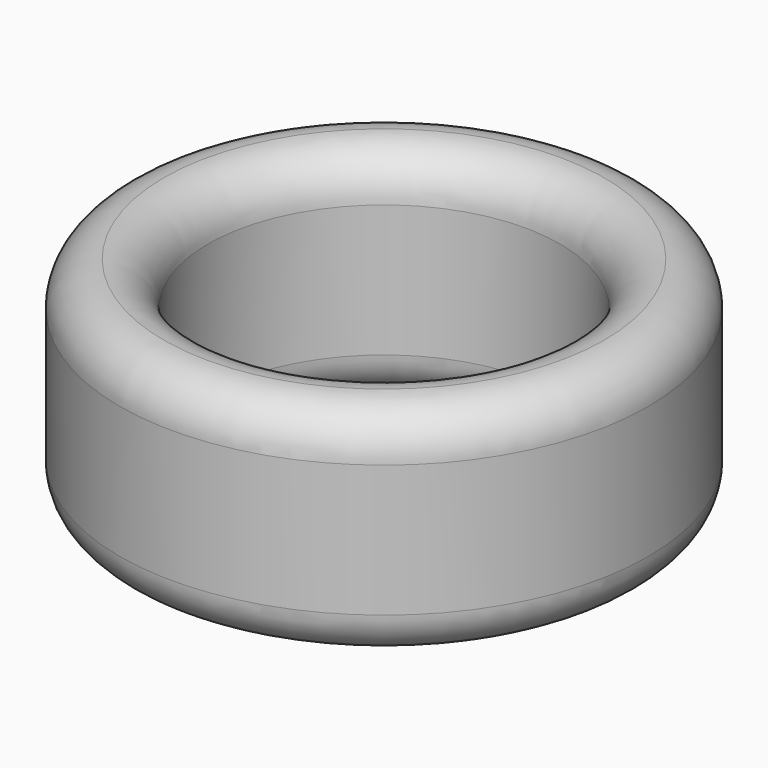
from build123d import *

# Parameters (mm, degrees)
F0_R     = 30
F0_R_2   = 20
F1_DEPTH = 25
F2_R     = 4.99999


# Not quite as in the source:
# - a fillet or chamfer is up to 0.001 mm smaller than in the source, because OpenCascade refuses the exact size


with BuildPart() as f1:
    # F0 (on Top) → F1 (new body)
    with BuildSketch(Plane.XY):
        Circle(F0_R)
        Circle(F0_R_2, mode=Mode.SUBTRACT)
    extrude(amount=F1_DEPTH)

    # F2 (radius 5 in the source; OpenCascade refuses exactly that, so slightly less here)
    f2_edges = [f1.edges().sort_by_distance(p)[0] for p in [
        (-30, 0, 25),
        (-20, 0, 25),
        (30, 0, 12.5),
        (-30, 0, 0),
        (-20, 0, 0),
    ]]
    fillet(f2_edges, radius=F2_R)


solid = f1.part
